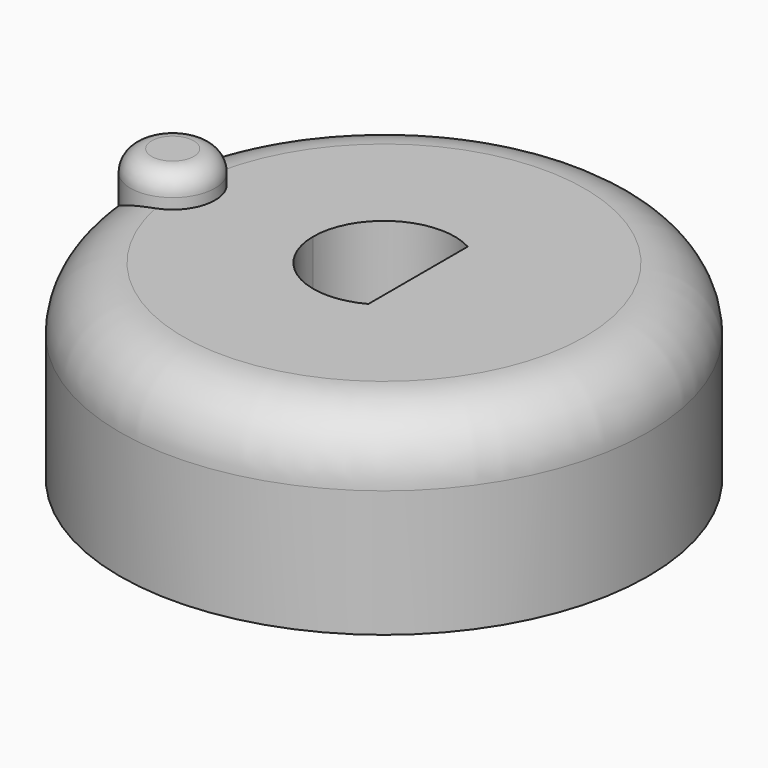
from build123d import *

# Parameters (mm, degrees)
F0_R        = 12.5
F1_DEPTH    = 9
F2_R        = 6.25
F3_DEPTH    = 4
F4_R        = 2
F5_DEPTH    = 1.5
F6_R        = 1
F7_S5_R     = 2
F7_T6_DEPTH = 21


# Not quite as in the source:
# - a fillet or chamfer that OpenCascade refuses, or shapes differently, is made with other operations: its cross-section is extruded or revolved along the edge and cut away or added


with BuildPart() as f1:
    # F0 (on Top) → F1 (new body)
    with BuildSketch(Plane.XY):
        Circle(F0_R)
        with BuildLine():
            ThreePointArc((-3.35, 0), (-1.7058759905, 2.8831384124), (1.6126788687, 2.9362845343))
            Line((1.6126788687, 2.9362845343), (1.6126788687, 0))
            Line((1.6126788687, 0), (1.6126788687, -2.9362845343))
            ThreePointArc((1.6126788687, -2.9362845343), (-1.7058759905, -2.8831384124), (-3.35, 0))
        make_face(mode=Mode.SUBTRACT)
    extrude(amount=F1_DEPTH)

    # F2 (on face) → F3 (cut)
    with BuildSketch(Plane(origin=(0, 0, 0), x_dir=(1, 0, 0), z_dir=(0, 0, -1))):
        with Locations((0, -0.4813171179)):
            Circle(F2_R)
    extrude(amount=-F3_DEPTH, mode=Mode.SUBTRACT)

    # F4 (on face) → F5 (join)
    with BuildSketch(Plane.XY.offset(9)):
        with Locations((-10, 0)):
            Circle(F4_R)
    extrude(amount=F5_DEPTH)

    # F6
    f6_edges = [f1.edges().sort_by_distance(p)[0] for p in [
        (-12, 0, 10.5),
    ]]
    fillet(f6_edges, radius=F6_R)

    # F7: fillet of radius 3 on 1 edges, made by hand


with BuildPart() as f7_tool2:
    # F7_s3 → F7_t4 (revolve)
    with BuildSketch(Plane.XZ):
        with BuildLine():
            ThreePointArc((9.5, 9), (11.6213203436, 8.1213203436), (12.5, 6))
            Line((12.5, 6), (12.5, 9))
            Line((12.5, 9), (9.5, 9))
        make_face()
    revolve(axis=Axis((0, 0, 9), (0, 0, 1)))

    # F7_s5 → F7_t6 (cut, symmetric)
    with BuildSketch(Plane.XY.offset(6.4)):
        with Locations((-10, 0)):
            Circle(F7_S5_R)
    extrude(amount=F7_T6_DEPTH, both=True, mode=Mode.SUBTRACT)


with BuildPart() as f1_1:
    add(f1.part)

    # F7_t1: cut F7_tool2
    add(f7_tool2.part, mode=Mode.SUBTRACT)


solid = f1_1.part
